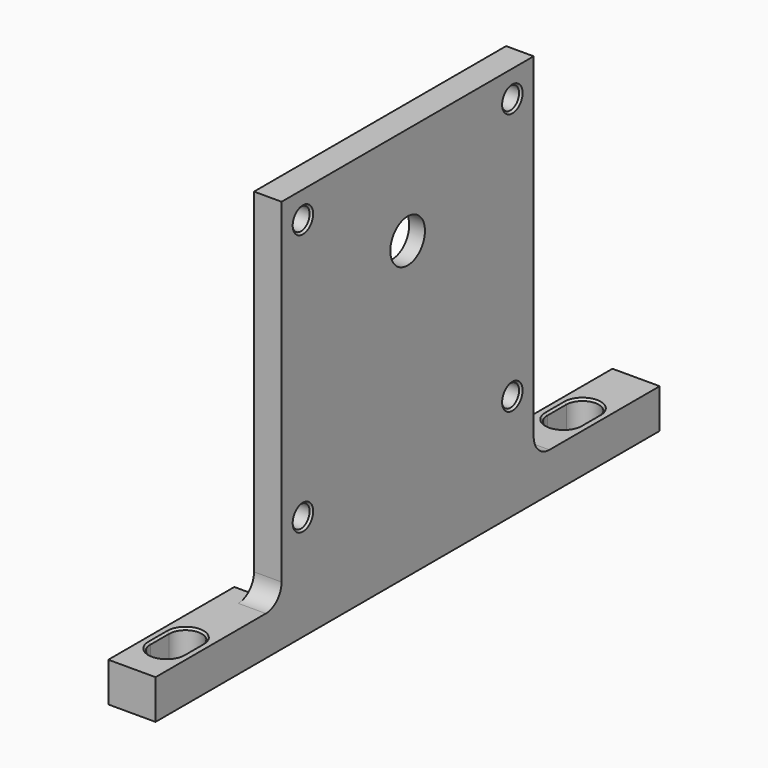
from build123d import *

# Parameters (mm, degrees)
F0_R      = 2.75
F1_DEPTH  = 12
F3_DEPTH  = 10.001
F4_SIZE   = 0.5
F5_SIZE   = 0.5
F6_W      = 80
F6_H      = 104
F7_DEPTH  = 5
F8_R      = 17
F8_R_2    = 5.5
F9_DEPTH  = 3
F10_R     = 5
F11_DEPTH = 7.001


with BuildPart() as f1:
    # F0 (on Right) → F1 (new body)
    with BuildSketch(Plane.YZ):
        Polygon((-80, 0), (0, 0), (80, 0), (80, 10), (40, 10), (40, 100), (0, 100), (-40, 100), (-40, 10), (-80, 10), align=None)
        with Locations((-33.2340187158, 26.7659812842)):
            Circle(F0_R, mode=Mode.SUBTRACT)
        with Locations((33.2340187158, 26.7659812842)):
            Circle(F0_R, mode=Mode.SUBTRACT)
        with Locations((-33.2340187158, 93.2340187158)):
            Circle(F0_R, mode=Mode.SUBTRACT)
        with Locations((33.2340187158, 93.2340187158)):
            Circle(F0_R, mode=Mode.SUBTRACT)
    extrude(amount=F1_DEPTH)

    # F2 (on face) → F3 (cut, through all)
    with BuildSketch(Plane.XY.offset(10)):
        with BuildLine():
            Line((10.125, 57), (10.125, 63))
            ThreePointArc((10.125, 63), (6, 67.125), (1.875, 63))
            Line((1.875, 63), (1.875, 57))
            ThreePointArc((1.875, 57), (6, 52.875), (10.125, 57))
        make_face()
        with BuildLine():
            Line((10.125, -69), (10.125, -63))
            ThreePointArc((10.125, -63), (6, -58.875), (1.875, -63))
            Line((1.875, -63), (1.875, -69))
            ThreePointArc((1.875, -69), (6, -73.125), (10.125, -69))
        make_face()
    extrude(amount=-F3_DEPTH, mode=Mode.SUBTRACT)

    # F4
    f4_edges = [f1.edges().sort_by_distance(p)[0] for p in [
        (6, 52.875, 10),
        (10.125, 57, 5),
        (6, 52.875, 0),
        (1.875, 57, 5),
        (6, -58.875, 10),
        (1.875, -63, 5),
        (6, -58.875, 0),
        (10.125, -63, 5),
    ]]
    chamfer(f4_edges, length=F4_SIZE)

    # F5
    f5_edges = [f1.edges().sort_by_distance(p)[0] for p in [
        (6, -30.484019, 93.234019),
        (0, -35.984019, 93.234019),
        (12, -35.984019, 93.234019),
        (6, 35.984019, 93.234019),
        (0, 30.484019, 93.234019),
        (12, 30.484019, 93.234019),
        (6, -30.484019, 26.765981),
        (0, -35.984019, 26.765981),
        (12, -35.984019, 26.765981),
        (6, 35.984019, 26.765981),
        (0, 30.484019, 26.765981),
        (12, 30.484019, 26.765981),
    ]]
    chamfer(f5_edges, length=F5_SIZE)

    # F6 (on face) → F7 (cut)
    with BuildSketch(Plane(origin=(0, 0, 0), x_dir=(0, -1, 0), z_dir=(-1, 0, 0))):
        with Locations((0, 48)):
            Rectangle(F6_W, F6_H)
    extrude(amount=-F7_DEPTH, mode=Mode.SUBTRACT)

    # F8 (on face) → F9 (cut)
    with BuildSketch(Plane(origin=(5, 0, 0), x_dir=(0, -1, 0), z_dir=(-1, 0, 0))):
        with Locations((0, 75)):
            Circle(F8_R)
        with Locations((0, 75)):
            Circle(F8_R_2, mode=Mode.SUBTRACT)
    extrude(amount=-F9_DEPTH, mode=Mode.SUBTRACT)

    # F10
    f10_edges = [f1.edges().sort_by_distance(p)[0] for p in [
        (8.5, 40, 10),
        (8.5, -40, 10),
    ]]
    fillet(f10_edges, radius=F10_R)

    # F11 (cut, through all): a face of the model
    f11_faces = [f1.faces().sort_by_distance(p)[0] for p in [
        (5, 0, 75),
    ]]
    extrude(f11_faces, amount=-F11_DEPTH, mode=Mode.SUBTRACT)


solid = f1.part
